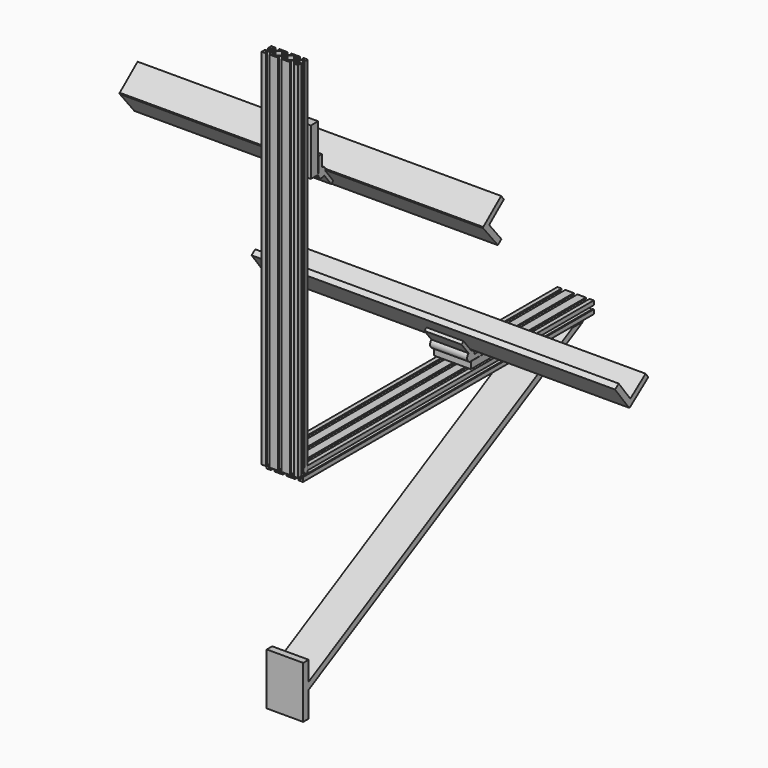
from build123d import *

# Parameters (mm, degrees)
F0_R          = 2.1
F1_DEPTH      = 600
F2_R          = 2.1
F3_DEPTH      = 600
F5_DEPTH      = 40.386
F5_DEPTH_BACK = 19.812
F6_W          = 67.6259994507
F6_H          = 11.4020574838
F7_DEPTH      = 40.64
F7_DEPTH_BACK = 20.574
F6_W_2        = 15.0790625318
F6_H_2        = 77.6842328595
F9_DEPTH      = 300
F9_DEPTH_BACK = 300


with BuildPart() as f1:
    # F0 (on Front) → F1 (new body)
    with BuildSketch(Plane.XZ):
        Polygon((16, -10), (20, -10), (21, -10), (27, -10), (27, -8), (23, -8), (28, -3), (32, -3), (36, -7), (36, -8), (33, -8), (33, -10), (36, -10), (40, -10), (40, -6), (40, -3), (38, -3), (38, -6), (37, -6), (33, -2), (33, 2), (37, 6), (38, 6), (38, 3), (40, 3), (40, 6), (40, 7.62), (40, 10), (39, 10), (36, 10), (33, 10), (33, 8), (36, 8), (36, 7), (32, 3), (28, 3), (23, 8), (27, 8), (27, 10), (20, 10), (16, 10), (13, 10), (13, 8), (16, 8), (17, 8), (12, 3), (8, 3), (3, 8), (4, 8), (7, 8), (7, 10), (1, 10), (0, 10), (-7, 10), (-7, 8), (-3, 8), (-8, 3), (-12, 3), (-16, 7), (-16, 8), (-13, 8), (-13, 10), (-16, 10), (-19, 10), (-20, 10), (-20, 7.62), (-20, 6), (-20, 3), (-18, 3), (-18, 6), (-17, 6), (-13, 2), (-13, -2), (-17, -6), (-18, -6), (-18, -3), (-20, -3), (-20, -6), (-20, -10), (-16, -10), (-13, -10), (-13, -8), (-16, -8), (-16, -7), (-12, -3), (-8, -3), (-3, -8), (-7, -8), (-7, -10), (-1, -10), (0, -10), (7, -10), (7, -8), (3, -8), (8, -3), (12, -3), (17, -8), (16, -8), (13, -8), (13, -10), align=None)
        with Locations((-10, 0)):
            Circle(F0_R, mode=Mode.SUBTRACT)
        Polygon((-2, -7), (-7, -2), (-7, 2), (-2, 7), (-1, 8), (1, 8), (2, 7), (7, 2), (7, -2), (2, -7), (1, -8), (-1, -8), align=None, mode=Mode.SUBTRACT)
        with Locations((10, 0)):
            Circle(F0_R, mode=Mode.SUBTRACT)
        Polygon((18, -7), (13, -2), (13, 2), (18, 7), (19, 8), (21, 8), (22, 7), (27, 2), (27, -2), (22, -7), (21, -8), (19, -8), align=None, mode=Mode.SUBTRACT)
        with Locations((30, 0)):
            Circle(F0_R, mode=Mode.SUBTRACT)
    extrude(amount=-F1_DEPTH)

    # F2 (on Top) → F3 (join)
    with BuildSketch(Plane.XY):
        Polygon((16.0137486309, -10.2479457855), (20.0137486309, -10.2479457855), (21.0137486309, -10.2479457855), (27.0137486309, -10.2479457855), (27.0137486309, -8.2479457855), (23.0137486309, -8.2479457855), (28.0137486309, -3.2479457855), (32.0137486309, -3.2479457855), (36.0137486309, -7.2479457855), (36.0137486309, -8.2479457855), (33.0137486309, -8.2479457855), (33.0137486309, -10.2479457855), (36.0137486309, -10.2479457855), (40.0137486309, -10.2479457855), (40.0137486309, -6.2479457855), (40.0137486309, -3.2479457855), (38.0137486309, -3.2479457855), (38.0137486309, -6.2479457855), (37.0137486309, -6.2479457855), (33.0137486309, -2.2479457855), (33.0137486309, 1.7520542145), (37.0137486309, 5.7520542145), (38.0137486309, 5.7520542145), (38.0137486309, 2.7520542145), (40.0137486309, 2.7520542145), (40.0137486309, 5.7520542145), (40.0137486309, 7.3720542145), (40.0137486309, 9.7520542145), (39.0137486309, 9.7520542145), (36.0137486309, 9.7520542145), (33.0137486309, 9.7520542145), (33.0137486309, 7.7520542145), (36.0137486309, 7.7520542145), (36.0137486309, 6.7520542145), (32.0137486309, 2.7520542145), (28.0137486309, 2.7520542145), (23.0137486309, 7.7520542145), (27.0137486309, 7.7520542145), (27.0137486309, 9.7520542145), (20.0137486309, 9.7520542145), (16.0137486309, 9.7520542145), (13.0137486309, 9.7520542145), (13.0137486309, 7.7520542145), (16.0137486309, 7.7520542145), (17.0137486309, 7.7520542145), (12.0137486309, 2.7520542145), (8.0137486309, 2.7520542145), (3.0137486309, 7.7520542145), (4.0137486309, 7.7520542145), (7.0137486309, 7.7520542145), (7.0137486309, 9.7520542145), (1.0137486309, 9.7520542145), (0.0137486309, 9.7520542145), (-6.9862513691, 9.7520542145), (-6.9862513691, 7.7520542145), (-2.9862513691, 7.7520542145), (-7.9862513691, 2.7520542145), (-11.9862513691, 2.7520542145), (-15.9862513691, 6.7520542145), (-15.9862513691, 7.7520542145), (-12.9862513691, 7.7520542145), (-12.9862513691, 9.7520542145), (-15.9862513691, 9.7520542145), (-18.9862513691, 9.7520542145), (-19.9862513691, 9.7520542145), (-19.9862513691, 7.3720542145), (-19.9862513691, 5.7520542145), (-19.9862513691, 2.7520542145), (-17.9862513691, 2.7520542145), (-17.9862513691, 5.7520542145), (-16.9862513691, 5.7520542145), (-12.9862513691, 1.7520542145), (-12.9862513691, -2.2479457855), (-16.9862513691, -6.2479457855), (-17.9862513691, -6.2479457855), (-17.9862513691, -3.2479457855), (-19.9862513691, -3.2479457855), (-19.9862513691, -6.2479457855), (-19.9862513691, -10.2479457855), (-15.9862513691, -10.2479457855), (-12.9862513691, -10.2479457855), (-12.9862513691, -8.2479457855), (-15.9862513691, -8.2479457855), (-15.9862513691, -7.2479457855), (-11.9862513691, -3.2479457855), (-7.9862513691, -3.2479457855), (-2.9862513691, -8.2479457855), (-6.9862513691, -8.2479457855), (-6.9862513691, -10.2479457855), (-0.9862513691, -10.2479457855), (0.0137486309, -10.2479457855), (7.0137486309, -10.2479457855), (7.0137486309, -8.2479457855), (3.0137486309, -8.2479457855), (8.0137486309, -3.2479457855), (12.0137486309, -3.2479457855), (17.0137486309, -8.2479457855), (16.0137486309, -8.2479457855), (13.0137486309, -8.2479457855), (13.0137486309, -10.2479457855), align=None)
        with Locations((-9.9862513691, -0.2479457855)):
            Circle(F2_R, mode=Mode.SUBTRACT)
        Polygon((-1.9862513691, -7.2479457855), (-6.9862513691, -2.2479457855), (-6.9862513691, 1.7520542145), (-1.9862513691, 6.7520542145), (-0.9862513691, 7.7520542145), (1.0137486309, 7.7520542145), (2.0137486309, 6.7520542145), (7.0137486309, 1.7520542145), (7.0137486309, -2.2479457855), (2.0137486309, -7.2479457855), (1.0137486309, -8.2479457855), (-0.9862513691, -8.2479457855), align=None, mode=Mode.SUBTRACT)
        with Locations((10.0137486309, -0.2479457855)):
            Circle(F2_R, mode=Mode.SUBTRACT)
        Polygon((18.0137486309, -7.2479457855), (13.0137486309, -2.2479457855), (13.0137486309, 1.7520542145), (18.0137486309, 6.7520542145), (19.0137486309, 7.7520542145), (21.0137486309, 7.7520542145), (22.0137486309, 6.7520542145), (27.0137486309, 1.7520542145), (27.0137486309, -2.2479457855), (22.0137486309, -7.2479457855), (21.0137486309, -8.2479457855), (19.0137486309, -8.2479457855), align=None, mode=Mode.SUBTRACT)
        with Locations((30.0137486309, -0.2479457855)):
            Circle(F2_R, mode=Mode.SUBTRACT)
    extrude(amount=F3_DEPTH)


with BuildPart() as f5:
    # F4 (on Right) → F5 (new body, two sides)
    with BuildSketch(Plane.YZ) as f5_sk:
        Polygon((577.4232465298, -11.5676193306), (577.0964622498, -11.5676193306), (577.0964622498, -11.7435521713), align=None)
        Polygon((577.0964622498, -11.7435521713), (577.0964622498, -11.5676193306), (555.6103307278, -11.5676193306), (11.2802451476, -304.6219187382), (11.2802451476, -291.0836935043), (11.2802451476, -272.7263271809), (0, -272.7263271809), (0, -291.0836935043), (0, -310.6949329376), (0, -322.4384851089), (0, -358.4799766541), (11.2802451476, -358.4799766541), (11.2802451476, -316.3654709095), align=None)
    extrude(amount=F5_DEPTH)
    extrude(f5_sk.sketch, amount=-F5_DEPTH_BACK)


with BuildPart() as f7:
    # F6 (on Right) → F7 (new body, two sides)
    with BuildSketch(Plane.YZ) as f7_sk:
        with Locations((379.4575035572, 19.3334678188)):
            Rectangle(F6_W, F6_H)
    extrude(amount=F7_DEPTH)
    extrude(f7_sk.sketch, amount=-F7_DEPTH_BACK)


with BuildPart() as f7b:
    # F6 (on Right) → F7, piece 2 (new body, two sides)
    with BuildSketch(Plane.YZ) as f7_2_sk:
        with BuildLine():
            ThreePointArc((340.9104562797, 38.732160941), (338.3981734553, 30.1969923926), (345.6445038319, 25.0344965607))
            ThreePointArc((345.6445038319, 25.0344965607), (346.6697853367, 25.1033604136), (347.676648747, 25.3087149061))
            Line((347.676648747, 25.3087149061), (347.676648747, 32.701395452))
            Line((347.676648747, 32.701395452), (345.6445038319, 32.701395452))
            Line((345.6445038319, 32.701395452), (340.9104562797, 38.732160941))
        make_face()
        with BuildLine():
            Line((347.676648747, 32.701395452), (347.676648747, 25.3087149061))
            ThreePointArc((347.676648747, 25.3087149061), (351.742109436, 28.0537568574), (353.3114027232, 32.701395452))
            Line((353.3114027232, 32.701395452), (347.676648747, 32.701395452))
        make_face()
        with BuildLine():
            ThreePointArc((353.3114027232, 32.701395452), (351.742109436, 28.0537568574), (347.676648747, 25.3087149061))
            Line((347.676648747, 25.3087149061), (374.1813004017, 25.3087149061))
            Line((374.1813004017, 25.3087149061), (374.1813004017, 32.701395452))
            Line((374.1813004017, 32.701395452), (353.3114027232, 32.701395452))
        make_face()
        with BuildLine():
            Line((326.322950049, 57.3153771373), (340.9104562797, 38.732160941))
            ThreePointArc((340.9104562797, 38.732160941), (343.5315072845, 40.0713740274), (346.4639791391, 40.3243737959))
            Line((346.4639791391, 40.3243737959), (330.5324480624, 60.6197609345))
            Line((330.5324480624, 60.6197609345), (326.322950049, 57.3153771373))
        make_face()
        with BuildLine():
            ThreePointArc((346.4639791391, 40.3243737959), (343.5315072845, 40.0713740274), (340.9104562797, 38.732160941))
            Line((340.9104562797, 38.732160941), (345.6445038319, 32.701395452))
            Line((345.6445038319, 32.701395452), (347.676648747, 32.701395452))
            Line((347.676648747, 32.701395452), (353.3114027232, 32.701395452))
            ThreePointArc((353.3114027232, 32.701395452), (351.3481944325, 37.8247978511), (346.4639791391, 40.3243737959))
        make_face()
    extrude(amount=F7_DEPTH)
    extrude(f7_2_sk.sketch, amount=-F7_DEPTH_BACK)


with BuildPart() as f7c:
    # F6 (on Right) → F7, piece 3 (new body, two sides)
    with BuildSketch(Plane.YZ) as f7_3_sk:
        with BuildLine():
            Line((38.2286199435, 426.7386130083), (38.2286199435, 424.3225363208))
            Line((38.2286199435, 424.3225363208), (42.9626674957, 418.2917708318))
            ThreePointArc((42.9626674957, 418.2917708318), (44.8859979515, 420.5198193095), (45.8281406629, 423.3083255713))
            ThreePointArc((45.8281406629, 423.3083255713), (45.878655747, 423.8143131261), (45.8955188348, 424.3225363208))
            ThreePointArc((45.8955188348, 424.3225363208), (43.6499361402, 429.7438525176), (38.2286199435, 431.9894352122))
            Line((38.2286199435, 431.9894352122), (38.2286199435, 426.7386130083))
        make_face()
        with BuildLine():
            Line((42.9626674957, 418.2917708318), (38.2286199435, 424.3225363208))
            Line((38.2286199435, 424.3225363208), (38.2286199435, 426.7386130083))
            Line((38.2286199435, 426.7386130083), (30.9523632101, 426.7386130083))
            ThreePointArc((30.9523632101, 426.7386130083), (30.6600116404, 425.5462629912), (30.5617210522, 424.3225363208))
            ThreePointArc((30.5617210522, 424.3225363208), (34.8755709817, 417.4277265867), (42.9626674957, 418.2917708318))
        make_face()
        with BuildLine():
            ThreePointArc((45.8281406629, 423.3083255713), (44.8859979515, 420.5198193095), (42.9626674957, 418.2917708318))
            Line((42.9626674957, 418.2917708318), (57.5501737264, 399.7085546355))
            Line((57.5501737264, 399.7085546355), (61.7596717397, 403.0129384327))
            Line((61.7596717397, 403.0129384327), (45.8281406629, 423.3083255713))
        make_face()
        with BuildLine():
            Line((30.9523632101, 426.7386130083), (38.2286199435, 426.7386130083))
            Line((38.2286199435, 426.7386130083), (38.2286199435, 431.9894352122))
            ThreePointArc((38.2286199435, 431.9894352122), (33.7421111152, 430.5396560031), (30.9523632101, 426.7386130083))
        make_face()
        with BuildLine():
            ThreePointArc((30.9523632101, 426.7386130083), (33.7421111152, 430.5396560031), (38.2286199435, 431.9894352122))
            Line((38.2286199435, 431.9894352122), (38.2286199435, 451.1919021606))
            Line((38.2286199435, 451.1919021606), (30.9523632101, 451.1919021606))
            Line((30.9523632101, 451.1919021606), (30.9523632101, 426.7386130083))
        make_face()
    extrude(amount=F7_DEPTH)
    extrude(f7_3_sk.sketch, amount=-F7_DEPTH_BACK)


with BuildPart() as f7d:
    # F6 (on Right) → F7, piece 4 (new body, two sides)
    with BuildSketch(Plane.YZ) as f7_4_sk:
        with Locations((23.0221897863, 463.1646527506)):
            Rectangle(F6_W_2, F6_H_2)
    extrude(amount=F7_DEPTH)
    extrude(f7_4_sk.sketch, amount=-F7_DEPTH_BACK)


with BuildPart() as f9:
    # F8 (on Right) → F9 (new body, two sides)
    with BuildSketch(Plane.YZ) as f9_sk:
        Polygon((46.9310618937, 426.0134952692), (46.9310618937, 424.1959154606), (77.1296024323, 387.3319327831), (84.4074771326, 393.2938820412), (59.1799772639, 424.0896126151), (89.6657304769, 449.0631826796), (83.8036795212, 456.2191094571), align=None)
    extrude(amount=F9_DEPTH)
    extrude(f9_sk.sketch, amount=-F9_DEPTH_BACK)


with BuildPart() as f9b:
    # F8 (on Right) → F9, piece 2 (new body, two sides)
    with BuildSketch(Plane.YZ) as f9_2_sk:
        Polygon((347.5880919454, 41.1849674582), (349.3536787328, 40.7533430187), (387.4514590367, 69.3982063469), (381.8923054501, 76.7919023681), (350.3936052483, 53.1087388058), (326.4696326599, 84.9277159546), (318.9499367649, 79.2738258995), align=None)
    extrude(amount=F9_DEPTH)
    extrude(f9_2_sk.sketch, amount=-F9_DEPTH_BACK)


solid = Compound([f1.part, f5.part, f7.part, f7b.part, f7c.part, f7d.part, f9.part, f9b.part])
